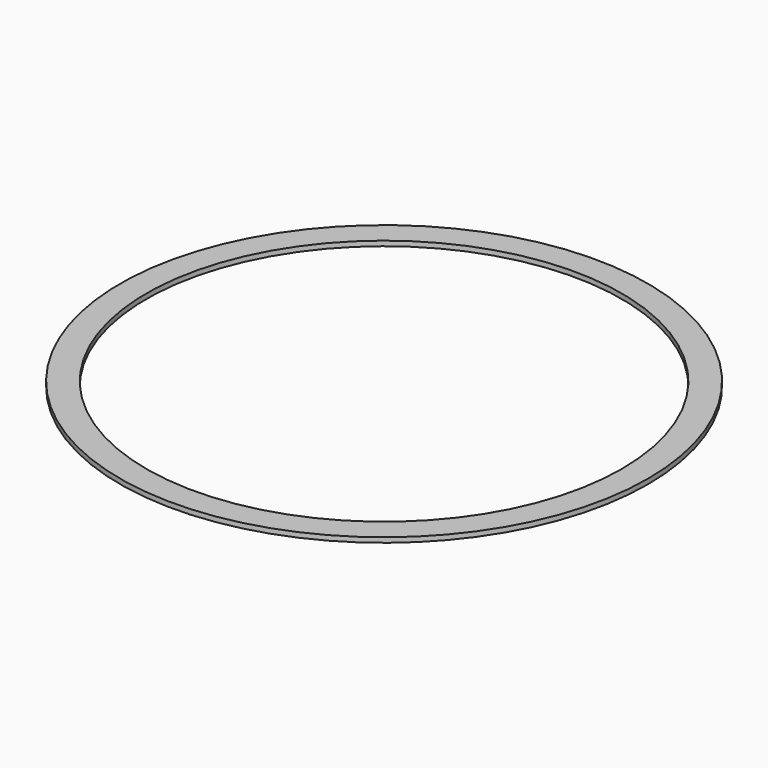
from build123d import *

# Parameters (mm, degrees)
F0_R     = 255.15443
F0_R_2   = 229.75443
F1_DEPTH = 4.7625


# Not quite as in the source:
# - a length typed as a fraction of an inch, garbled in the dataset ("3 / 203.2 mm" for 3/8 in), is restored


with BuildPart() as f1:
    # F0 (on Top) → F1 (new body)
    with BuildSketch(Plane.XY):
        Circle(F0_R)
        Circle(F0_R_2, mode=Mode.SUBTRACT)
    extrude(amount=F1_DEPTH)


solid = f1.part
